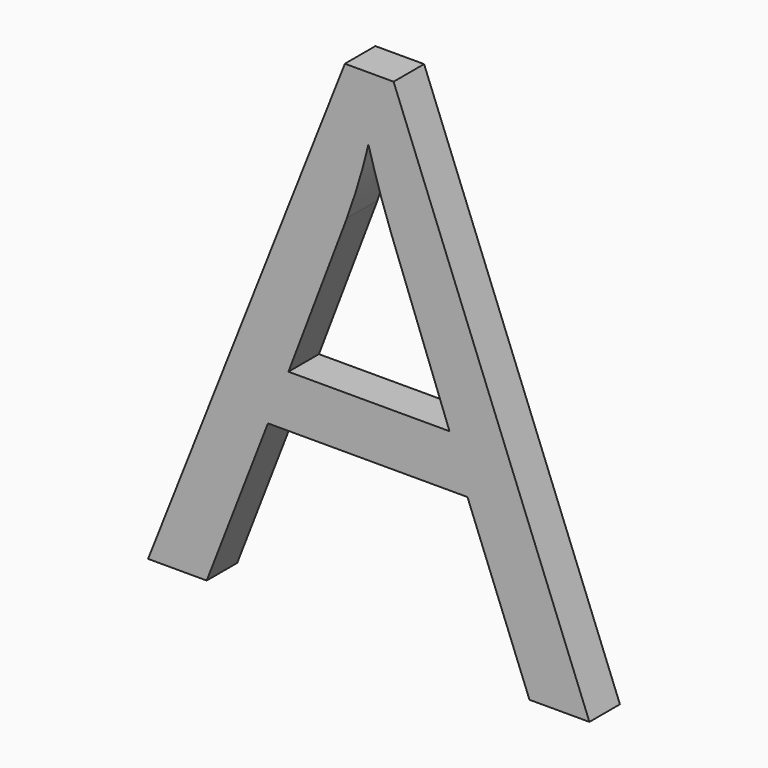
from build123d import *

# Parameters (mm, degrees)
F0_TEXT_SIZE = 46.4434631997
F1_DEPTH     = 2.54


# Not quite as in the source:
# - Text() gives the source's letters only with a copy of the font that has no kerning and outlines rounded to 1/6400 em; it was checked with that copy


with BuildPart() as f1:
    # F0 (on Front) → F1 (new body)
    with BuildSketch(Plane.XZ):
        with Locations((-32.4015723729, 0)):
            Text('A', F0_TEXT_SIZE, font='Open Sans', text_align=(TextAlign.LEFT, TextAlign.BOTTOM))
    extrude(amount=F1_DEPTH)


solid = f1.part
